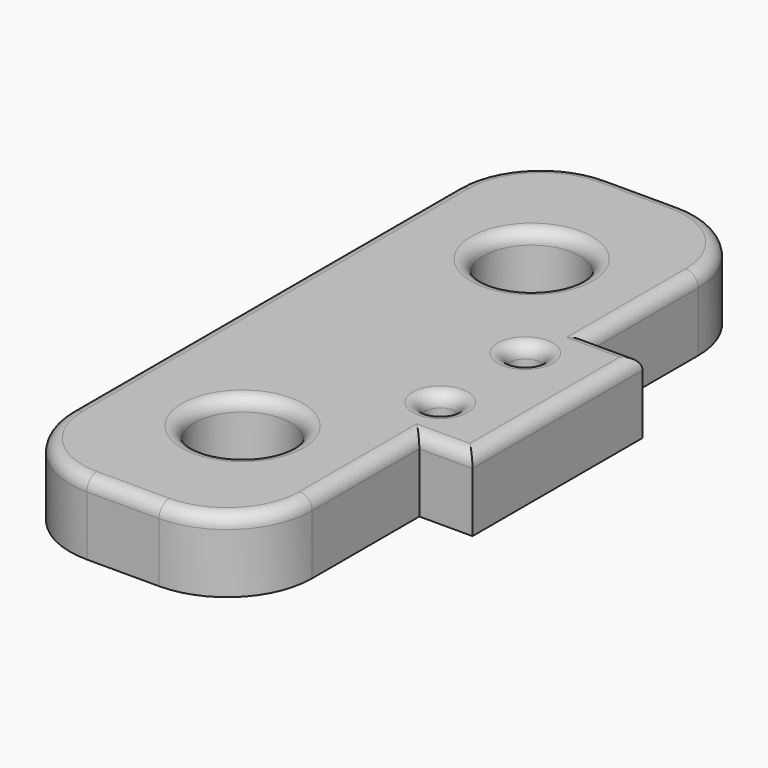
from build123d import *

# Parameters (mm, degrees)
F0_R     = 2.8575
F0_R_2   = 0.889
F0_R_3   = 1.905
F0_R_4   = 11.7475
F1_DEPTH = 4.318
F2_W     = 12.7
F2_H     = 4.318
F3_DEPTH = 3.175
F4_R     = 5.08
F6_DEPTH = 25.4
F7_R     = 5.08
F8_R     = 0.762


# Not quite as in the source:
# - a feature names something its author has since deleted; it is built from what else it names


with BuildPart() as f1:
    # F0 (on Top) → F1 (new body)
    with BuildSketch(Plane.XY):
        Polygon((0, -20.7006), (0, 0), (0, 63.5), (-41.91, 63.5), (-41.91, 19), (-41.91, 0), (-41.91, -20.7006), align=None)
        with Locations((-34.925, -12.09)):
            Circle(F0_R, mode=Mode.SUBTRACT)
        with Locations((-34.925, 9.5)):
            Circle(F0_R, mode=Mode.SUBTRACT)
        with Locations((-6.985, -12.09)):
            Circle(F0_R, mode=Mode.SUBTRACT)
        with Locations((-1.27, -4.47)):
            Circle(F0_R_2, mode=Mode.SUBTRACT)
        with Locations((-6.985, 9.5)):
            Circle(F0_R, mode=Mode.SUBTRACT)
        with Locations((-1.27, 1.88)):
            Circle(F0_R_2, mode=Mode.SUBTRACT)
        with Locations((-36.83, 27.178)):
            Circle(F0_R_3, mode=Mode.SUBTRACT)
        with Locations((-36.83, 58.293)):
            Circle(F0_R_3, mode=Mode.SUBTRACT)
        with Locations((-5.08, 27.178)):
            Circle(F0_R_3, mode=Mode.SUBTRACT)
        with Locations((-20.955, 42.7355)):
            Circle(F0_R_4, mode=Mode.SUBTRACT)
        with Locations((-5.08, 58.293)):
            Circle(F0_R_3, mode=Mode.SUBTRACT)
    extrude(amount=F1_DEPTH)

    # F2 (on face) → F3 (join)
    with BuildSketch(Plane.YZ):
        with Locations((-1.2696, 2.159)):
            Rectangle(F2_W, F2_H)
    extrude(amount=F3_DEPTH)

    # F4
    f4_edges = [f1.edges().sort_by_distance(p)[0] for p in [
        (0, 63.5, 2.159),
        (-41.91, 63.5, 2.159),
        (0, -20.7006, 2.159),
        (-41.91, -20.7006, 2.159),
    ]]
    fillet(f4_edges, radius=F4_R)

    # F5 (on face) → F6 (cut)
    with BuildSketch(Plane.XY.offset(4.318)):
        Polygon((-51.067360534, -23.478101939), (-14.478, -25.962697342), (-14.478, 18.2829182773), (4.9410860353, 18.2829182773), (4.9410860353, 69.2363290038), (-51.067360534, 69.2363290038), align=None)
    extrude(amount=-F6_DEPTH, mode=Mode.SUBTRACT)

    # F7
    f7_edges = [f1.edges().sort_by_distance(p)[0] for p in [
        (-14.478, -20.7006, 2.159),
        (-14.478, 18.282918, 2.159),
        (0, 18.282918, 2.159),
    ]]
    fillet(f7_edges, radius=F7_R)

    # F8
    f8_edges = [f1.edges().sort_by_distance(p)[0] for p in [
        (0, 9.141659, 4.318),
        (-1.487898, 16.795021, 4.318),
        (1.5875, 5.0804, 4.318),
        (-7.239, 18.282918, 4.318),
        (3.175, -1.2696, 4.318),
        (-12.990102, 16.795021, 4.318),
        (1.5875, -7.6196, 4.318),
        (-14.478, -1.208841, 4.318),
        (0, -11.6201, 4.318),
        (-12.990102, -19.212702, 4.318),
        (-1.487898, -19.212702, 4.318),
        (-7.239, -20.7006, 4.318),
        (-9.8425, -12.09, 4.318),
        (-2.159, -4.47, 4.318),
        (-2.159, 1.88, 4.318),
        (-9.8425, 9.5, 4.318),
    ]]
    fillet(f8_edges, radius=F8_R)


solid = f1.part
